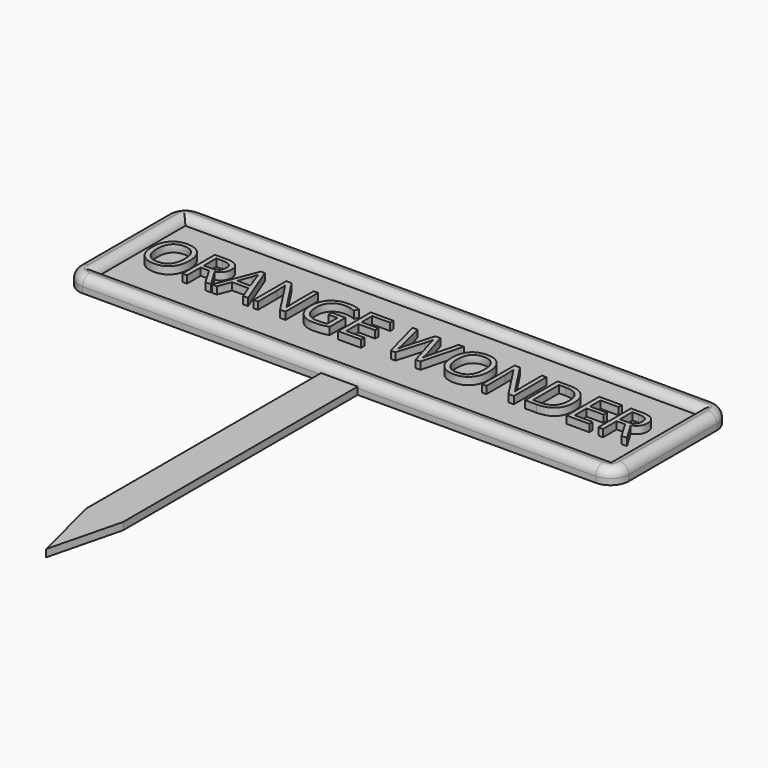
from build123d import *

# Parameters (mm, degrees)
F1_DEPTH     = 1
F2_W         = 70
F2_H         = 15
F2_TEXT_SIZE = 7.782964036
F3_DEPTH     = 1
F4_T1_DEPTH  = 15
F4_T3_DEPTH  = 70
F4_T8_DEPTH  = 70
F4_T13_DEPTH = 70
F4_T18_DEPTH = 70
F4_T21_ANGLE = 90
F4_T23_ANGLE = 90
F4_T25_ANGLE = 90
F4_T27_ANGLE = 90
F4_T32_DEPTH = 17.9580398916
F4_S33_R     = 2.5
F4_T34_DEPTH = 11
F4_T38_DEPTH = 72.9580398916
F4_S39_R     = 2.5
F4_T40_DEPTH = 38
F4_T47_DEPTH = 17.9580398916
F4_S48_R     = 2.5
F4_T49_DEPTH = 11
F4_T53_DEPTH = 72.9580398916
F4_S54_R     = 2.5
F4_T55_DEPTH = 38
F4_T62_DEPTH = 72.9580398916
F4_S64_R     = 2.5
F4_T65_DEPTH = 38
F4_T68_DEPTH = 17.9580398916
F4_S70_R     = 2.5
F4_T71_DEPTH = 11
F4_T77_DEPTH = 17.9580398916
F4_S78_R     = 2.5
F4_T79_DEPTH = 11
F4_T83_DEPTH = 72.9580398916
F4_S84_R     = 2.5
F4_T85_DEPTH = 38


# Not quite as in the source:
# - a fillet or chamfer that OpenCascade refuses, or shapes differently, is made with other operations: its cross-section is extruded or revolved along the edge and cut away or added
# - Text() gives the source's letters only with a copy of the font that has no kerning and outlines rounded to 1/6400 em; it was checked with that copy


with BuildPart() as f1:
    # F0 (on Top) → F1 (new body)
    with BuildSketch(Plane.XY):
        with BuildLine():
            Line((2.5, -10), (35, -10))
            ThreePointArc((35, -10), (36.767766953, -9.267766953), (37.5, -7.5))
            Line((37.5, -7.5), (37.5, 7.5))
            ThreePointArc((37.5, 7.5), (36.767766953, 9.267766953), (35, 10))
            Line((35, 10), (-35, 10))
            ThreePointArc((-35, 10), (-36.767766953, 9.267766953), (-37.5, 7.5))
            Line((-37.5, 7.5), (-37.5, -7.5))
            ThreePointArc((-37.5, -7.5), (-36.767766953, -9.267766953), (-35, -10))
            Line((-35, -10), (-2.5, -10))
            Line((-2.5, -10), (-2.5, -50))
            Line((-2.5, -50), (0, -60))
            Line((0, -60), (2.5, -50))
            Line((2.5, -50), (2.5, -10))
        make_face()
    extrude(amount=F1_DEPTH)

    # F2 (on face) → F3 (join)
    with BuildSketch(Plane.XY.offset(1)):
        with BuildLine():
            Line((2.5, -10), (35, -10))
            ThreePointArc((35, -10), (36.767766953, -9.267766953), (37.5, -7.5))
            Line((37.5, -7.5), (37.5, 7.5))
            ThreePointArc((37.5, 7.5), (36.767766953, 9.267766953), (35, 10))
            Line((35, 10), (-35, 10))
            ThreePointArc((-35, 10), (-36.767766953, 9.267766953), (-37.5, 7.5))
            Line((-37.5, 7.5), (-37.5, -7.5))
            ThreePointArc((-37.5, -7.5), (-36.767766953, -9.267766953), (-35, -10))
            Line((-35, -10), (-2.5, -10))
            Line((-2.5, -10), (2.5, -10))
        make_face()
        Rectangle(F2_W, F2_H, mode=Mode.SUBTRACT)
        with Locations((-34, -2.801867053)):
            Text('ORANGE WONDER', F2_TEXT_SIZE, font='Open Sans', text_align=(TextAlign.LEFT, TextAlign.BOTTOM))
    extrude(amount=F3_DEPTH)

    # F4: fillet of radius 1.2 on 12 edges, made by hand

    # F4_s2 → F4_t1 (cut)
    with BuildSketch(Plane.XZ.offset(-7.5)):
        with BuildLine():
            ThreePointArc((37.5, 0.8), (37.1485281374, 1.6485281374), (36.3, 2))
            Line((36.3, 2), (37.5, 2))
            Line((37.5, 2), (37.5, 0.8))
        make_face()
        with BuildLine():
            ThreePointArc((-37.5, 0.8), (-37.1485281374, 1.6485281374), (-36.3, 2))
            Line((-36.3, 2), (-37.5, 2))
            Line((-37.5, 2), (-37.5, 0.8))
        make_face()
        with BuildLine():
            ThreePointArc((36.1832159566, 2), (35.4086192874, 1.716515139), (35, 1))
            Line((35, 1), (35, 2))
            Line((35, 2), (36.1832159566, 2))
        make_face()
        with BuildLine():
            ThreePointArc((-36.1832159566, 2), (-35.4086192874, 1.716515139), (-35, 1))
            Line((-35, 1), (-35, 2))
            Line((-35, 2), (-36.1832159566, 2))
        make_face()
    extrude(amount=F4_T1_DEPTH, mode=Mode.SUBTRACT)

    # F4_s4 → F4_t3 (cut)
    with BuildSketch(Plane.YZ.offset(-35)):
        with BuildLine():
            ThreePointArc((10, 0.8), (9.6485281374, 1.6485281374), (8.8, 2))
            Line((8.8, 2), (10, 2))
            Line((10, 2), (10, 0.8))
        make_face()
        with BuildLine():
            ThreePointArc((-8.6832159566, 2), (-7.9086192874, 1.716515139), (-7.5, 1))
            Line((-7.5, 1), (-7.5, 2))
            Line((-7.5, 2), (-8.6832159566, 2))
        make_face()
        with BuildLine():
            ThreePointArc((8.6832159566, 2), (7.9086192874, 1.716515139), (7.5, 1))
            Line((7.5, 1), (7.5, 2))
            Line((7.5, 2), (8.6832159566, 2))
        make_face()
    extrude(amount=F4_T3_DEPTH, mode=Mode.SUBTRACT)


with BuildPart() as f4_tool6:
    # F4_s7 → F4_t8 (new body)
    with BuildSketch(Plane.YZ.offset(-35)):
        with BuildLine():
            ThreePointArc((-10, 0.8), (-9.6485281374, 1.6485281374), (-8.8, 2))
            Line((-8.8, 2), (-10, 2))
            Line((-10, 2), (-10, 0.8))
        make_face()
    extrude(amount=F4_T8_DEPTH)

    split(bisect_by=Plane.YZ.offset(-2.5), keep=Keep.BOTTOM)


with BuildPart() as f1_1:
    add(f1.part)

    # F4_t5: cut F4_tool6
    add(f4_tool6.part, mode=Mode.SUBTRACT)


with BuildPart() as f4_tool11:
    # F4_s12 → F4_t13 (new body)
    with BuildSketch(Plane.YZ.offset(-35)):
        with BuildLine():
            ThreePointArc((-10, 0.8), (-9.6485281374, 1.6485281374), (-8.8, 2))
            Line((-8.8, 2), (-10, 2))
            Line((-10, 2), (-10, 0.8))
        make_face()
    extrude(amount=F4_T13_DEPTH)

    split(bisect_by=Plane.XY.offset(1), keep=Keep.TOP)


with BuildPart() as f1_2:
    add(f1_1.part)

    # F4_t10: cut F4_tool11
    add(f4_tool11.part, mode=Mode.SUBTRACT)


with BuildPart() as f4_tool16:
    # F4_s17 → F4_t18 (new body)
    with BuildSketch(Plane.YZ.offset(-35)):
        with BuildLine():
            ThreePointArc((-10, 0.8), (-9.6485281374, 1.6485281374), (-8.8, 2))
            Line((-8.8, 2), (-10, 2))
            Line((-10, 2), (-10, 0.8))
        make_face()
    extrude(amount=F4_T18_DEPTH)

    split(bisect_by=Plane.YZ.offset(2.5), keep=Keep.TOP)


with BuildPart() as f1_3:
    add(f1_2.part)

    # F4_t15: cut F4_tool16
    add(f4_tool16.part, mode=Mode.SUBTRACT)

    # F4_s20 → F4_t21 (revolve, cut)
    with BuildSketch(Plane.YZ.offset(35)):
        with BuildLine():
            ThreePointArc((-10, 0.8), (-9.6485281374, 1.6485281374), (-8.8, 2))
            Line((-8.8, 2), (-10, 2))
            Line((-10, 2), (-10, 0.8))
        make_face()
    revolve(axis=Axis((35, -7.5, 2), (0, 0, 1)), revolution_arc=F4_T21_ANGLE, mode=Mode.SUBTRACT)

    # F4_s22 → F4_t23 (revolve, cut)
    with BuildSketch(Plane.XZ.offset(-7.5)):
        with BuildLine():
            ThreePointArc((37.5, 0.8), (37.1485281374, 1.6485281374), (36.3, 2))
            Line((36.3, 2), (37.5, 2))
            Line((37.5, 2), (37.5, 0.8))
        make_face()
    revolve(axis=Axis((35, 7.5, 2), (0, 0, 1)), revolution_arc=F4_T23_ANGLE, mode=Mode.SUBTRACT)

    # F4_s24 → F4_t25 (revolve, cut)
    with BuildSketch(Plane.YZ.offset(-35)):
        with BuildLine():
            ThreePointArc((10, 0.8), (9.6485281374, 1.6485281374), (8.8, 2))
            Line((8.8, 2), (10, 2))
            Line((10, 2), (10, 0.8))
        make_face()
    revolve(axis=Axis((-35, 7.5, 2), (0, 0, 1)), revolution_arc=F4_T25_ANGLE, mode=Mode.SUBTRACT)

    # F4_s26 → F4_t27 (revolve, cut)
    with BuildSketch(Plane.XZ.offset(7.5)):
        with BuildLine():
            ThreePointArc((-36.3, 2), (-37.1485281374, 1.6485281374), (-37.5, 0.8))
            Line((-37.5, 0.8), (-37.5, 2))
            Line((-37.5, 2), (-36.3, 2))
        make_face()
    revolve(axis=Axis((-35, -7.5, 2), (0, 0, 1)), revolution_arc=F4_T27_ANGLE, mode=Mode.SUBTRACT)


with BuildPart() as f4_tool30:
    # F4_s31 → F4_t32 (new body)
    with BuildSketch(Plane.XZ.offset(-10.4580398916)):
        with BuildLine():
            ThreePointArc((36.1832159566, 2), (35.4086192874, 1.716515139), (35, 1))
            Line((35, 1), (35, 2))
            Line((35, 2), (36.1832159566, 2))
        make_face()
    extrude(amount=F4_T32_DEPTH)

    # F4_s33 → F4_t34 (intersect, symmetric)
    with BuildSketch(Plane.XY.offset(1.5)):
        with Locations((35, 7.5)):
            Circle(F4_S33_R)
    extrude(amount=F4_T34_DEPTH, both=True, mode=Mode.INTERSECT)

    split(bisect_by=Plane.XZ.offset(-7.5), keep=Keep.BOTTOM)


with BuildPart() as f4_tool36:
    # F4_s37 → F4_t38 (new body)
    with BuildSketch(Plane.YZ.offset(-35)):
        with BuildLine():
            ThreePointArc((8.6832159566, 2), (7.9086192874, 1.716515139), (7.5, 1))
            Line((7.5, 1), (7.5, 2))
            Line((7.5, 2), (8.6832159566, 2))
        make_face()
    extrude(amount=F4_T38_DEPTH)

    # F4_s39 → F4_t40 (intersect, symmetric)
    with BuildSketch(Plane.XY.offset(1.5)):
        with Locations((35, 7.5)):
            Circle(F4_S39_R)
    extrude(amount=F4_T40_DEPTH, both=True, mode=Mode.INTERSECT)

    split(bisect_by=Plane.YZ.offset(35), keep=Keep.TOP)


with BuildPart() as f4_tool30_1:
    add(f4_tool30.part)

    # F4_t42: intersect F4_tool36
    add(f4_tool36.part, mode=Mode.INTERSECT)


with BuildPart() as f1_4:
    add(f1_3.part)

    # F4_t28: cut F4_tool30
    add(f4_tool30_1.part, mode=Mode.SUBTRACT)


with BuildPart() as f4_tool45:
    # F4_s46 → F4_t47 (new body)
    with BuildSketch(Plane.XZ.offset(-7.5)):
        with BuildLine():
            ThreePointArc((36.1832159566, 2), (35.4086192874, 1.716515139), (35, 1))
            Line((35, 1), (35, 2))
            Line((35, 2), (36.1832159566, 2))
        make_face()
    extrude(amount=F4_T47_DEPTH)

    # F4_s48 → F4_t49 (intersect, symmetric)
    with BuildSketch(Plane.XY.offset(1.5)):
        with Locations((35, -7.5)):
            Circle(F4_S48_R)
    extrude(amount=F4_T49_DEPTH, both=True, mode=Mode.INTERSECT)

    split(bisect_by=Plane.XZ.offset(7.5), keep=Keep.TOP)


with BuildPart() as f4_tool51:
    # F4_s52 → F4_t53 (new body)
    with BuildSketch(Plane.YZ.offset(37.9580398916)):
        with BuildLine():
            ThreePointArc((-8.6832159566, 2), (-7.9086192874, 1.716515139), (-7.5, 1))
            Line((-7.5, 1), (-7.5, 2))
            Line((-7.5, 2), (-8.6832159566, 2))
        make_face()
    extrude(amount=-F4_T53_DEPTH)

    # F4_s54 → F4_t55 (intersect, symmetric)
    with BuildSketch(Plane.XY.offset(1.5)):
        with Locations((35, -7.5)):
            Circle(F4_S54_R)
    extrude(amount=F4_T55_DEPTH, both=True, mode=Mode.INTERSECT)

    split(bisect_by=Plane.YZ.offset(35), keep=Keep.TOP)


with BuildPart() as f4_tool45_1:
    add(f4_tool45.part)

    # F4_t57: intersect F4_tool51
    add(f4_tool51.part, mode=Mode.INTERSECT)


with BuildPart() as f1_5:
    add(f1_4.part)

    # F4_t43: cut F4_tool45
    add(f4_tool45_1.part, mode=Mode.SUBTRACT)


with BuildPart() as f4_tool60:
    # F4_s61 → F4_t62 (new body)
    with BuildSketch(Plane.YZ.offset(35)):
        with BuildLine():
            ThreePointArc((-8.6832159566, 2), (-7.9086192874, 1.716515139), (-7.5, 1))
            Line((-7.5, 1), (-7.5, 2))
            Line((-7.5, 2), (-8.6832159566, 2))
        make_face()
    extrude(amount=-F4_T62_DEPTH)

    split(bisect_by=Plane.YZ.offset(-35), keep=Keep.BOTTOM)

    # F4_s64 → F4_t65 (intersect, symmetric)
    with BuildSketch(Plane.XY.offset(1.5)):
        with Locations((-35, -7.5)):
            Circle(F4_S64_R)
    extrude(amount=F4_T65_DEPTH, both=True, mode=Mode.INTERSECT)


with BuildPart() as f4_tool66:
    # F4_s67 → F4_t68 (new body)
    with BuildSketch(Plane.XZ.offset(10.4580398916)):
        with BuildLine():
            ThreePointArc((-36.1832159566, 2), (-35.4086192874, 1.716515139), (-35, 1))
            Line((-35, 1), (-35, 2))
            Line((-35, 2), (-36.1832159566, 2))
        make_face()
    extrude(amount=-F4_T68_DEPTH)

    split(bisect_by=Plane.XZ.offset(7.5), keep=Keep.TOP)

    # F4_s70 → F4_t71 (intersect, symmetric)
    with BuildSketch(Plane.XY.offset(1.5)):
        with Locations((-35, -7.5)):
            Circle(F4_S70_R)
    extrude(amount=F4_T71_DEPTH, both=True, mode=Mode.INTERSECT)


with BuildPart() as f4_tool60_1:
    add(f4_tool60.part)

    # F4_t72: intersect F4_tool66
    add(f4_tool66.part, mode=Mode.INTERSECT)


with BuildPart() as f1_6:
    add(f1_5.part)

    # F4_t58: cut F4_tool60
    add(f4_tool60_1.part, mode=Mode.SUBTRACT)


with BuildPart() as f4_tool75:
    # F4_s76 → F4_t77 (new body)
    with BuildSketch(Plane.XZ.offset(7.5)):
        with BuildLine():
            ThreePointArc((-36.1832159566, 2), (-35.4086192874, 1.716515139), (-35, 1))
            Line((-35, 1), (-35, 2))
            Line((-35, 2), (-36.1832159566, 2))
        make_face()
    extrude(amount=-F4_T77_DEPTH)

    # F4_s78 → F4_t79 (intersect, symmetric)
    with BuildSketch(Plane.XY.offset(1.5)):
        with Locations((-35, 7.5)):
            Circle(F4_S78_R)
    extrude(amount=F4_T79_DEPTH, both=True, mode=Mode.INTERSECT)

    split(bisect_by=Plane.XZ.offset(-7.5), keep=Keep.BOTTOM)


with BuildPart() as f4_tool81:
    # F4_s82 → F4_t83 (new body)
    with BuildSketch(Plane.YZ.offset(-37.9580398916)):
        with BuildLine():
            ThreePointArc((8.6832159566, 2), (7.9086192874, 1.716515139), (7.5, 1))
            Line((7.5, 1), (7.5, 2))
            Line((7.5, 2), (8.6832159566, 2))
        make_face()
    extrude(amount=F4_T83_DEPTH)

    # F4_s84 → F4_t85 (intersect, symmetric)
    with BuildSketch(Plane.XY.offset(1.5)):
        with Locations((-35, 7.5)):
            Circle(F4_S84_R)
    extrude(amount=F4_T85_DEPTH, both=True, mode=Mode.INTERSECT)

    split(bisect_by=Plane.YZ.offset(-35), keep=Keep.BOTTOM)


with BuildPart() as f4_tool75_1:
    add(f4_tool75.part)

    # F4_t87: intersect F4_tool81
    add(f4_tool81.part, mode=Mode.INTERSECT)


with BuildPart() as f1_7:
    add(f1_6.part)

    # F4_t73: cut F4_tool75
    add(f4_tool75_1.part, mode=Mode.SUBTRACT)


solid = f1_7.part
